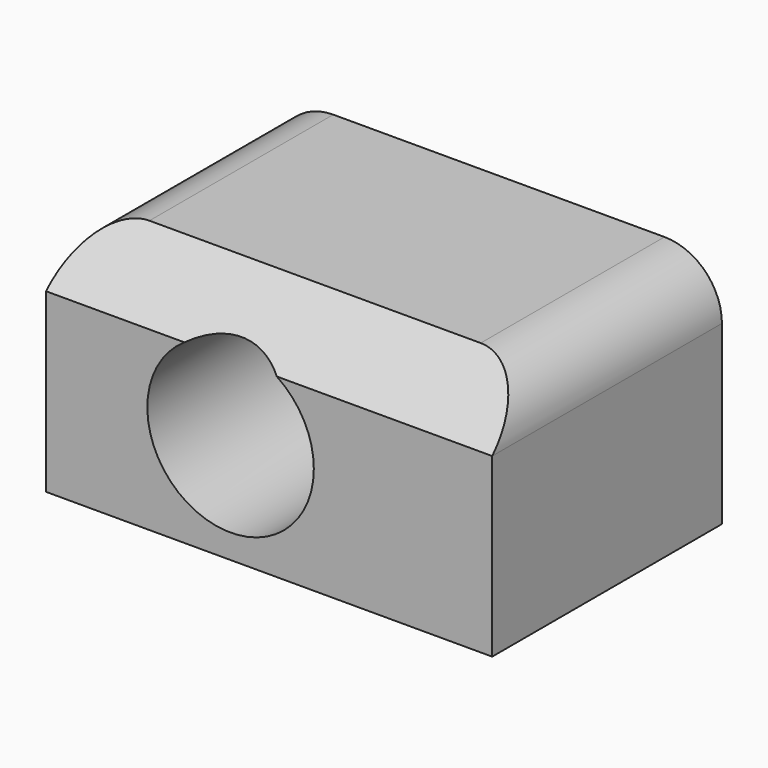
from build123d import *

# Parameters (mm, degrees)
F0_W        = 39.4569858909
F0_H        = 20.7027406432
F1_DEPTH    = 25.4
F2_R        = 7.3634612469
F3_DEPTH    = 25.4
F4_T1_DEPTH = 65.5852850486
F5_R        = 5.08
F6_R        = 5.08


# Not quite as in the source:
# - a fillet or chamfer that OpenCascade refuses, or shapes differently, is made with other operations: its cross-section is extruded or revolved along the edge and cut away or added


with BuildPart() as f1:
    # F0 (on Front) → F1 (new body)
    with BuildSketch(Plane.XZ):
        with Locations((-6.9415066391, 7.18506868)):
            Rectangle(F0_W, F0_H)
    extrude(amount=F1_DEPTH)

    # F2 (on face) → F3 (cut)
    with BuildSketch(Plane.XZ.offset(25.4)):
        with Locations((-10.3513691574, 6.3326032832)):
            Circle(F2_R)
    extrude(amount=-F3_DEPTH, mode=Mode.SUBTRACT)

    # F4: chamfer of 5.08 on 1 edges, made by hand

    # F4_s2 → F4_t1 (cut)
    with BuildSketch(Plane.YZ.offset(-39.7341491634)):
        Polygon((-20.32, 17.5364390016), (-25.4, 12.4564390016), (-25.4, 17.5364390016), align=None)
    extrude(amount=F4_T1_DEPTH, mode=Mode.SUBTRACT)

    # F5
    f5_edges = [f1.edges().sort_by_distance(p)[0] for p in [
        (12.786986, -10.16, 17.536439),
    ]]
    fillet(f5_edges, radius=F5_R)

    # F6
    f6_edges = [f1.edges().sort_by_distance(p)[0] for p in [
        (-26.67, -10.16, 17.536439),
    ]]
    fillet(f6_edges, radius=F6_R)


solid = f1.part
